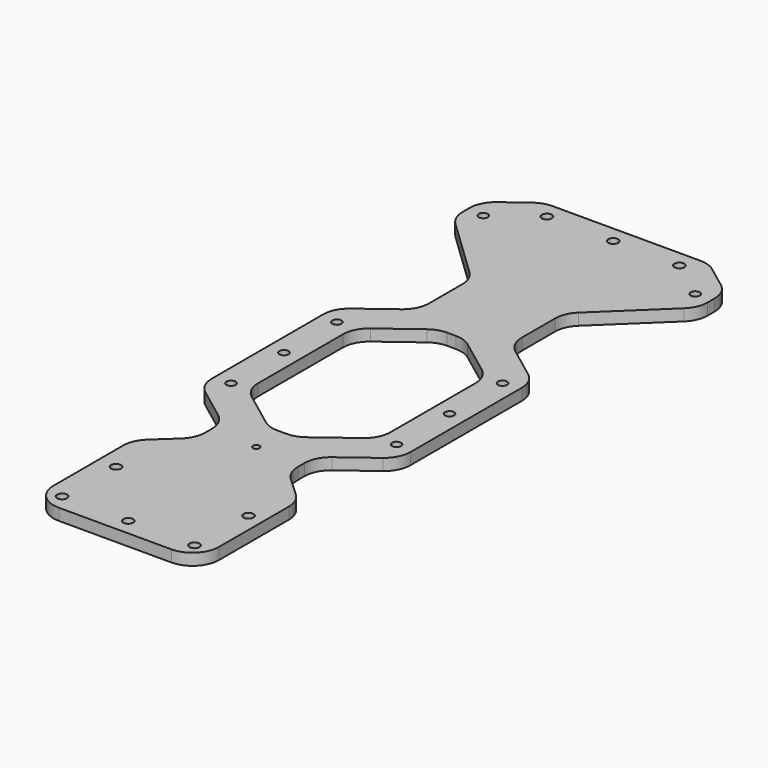
from build123d import *

# Parameters (mm, degrees)
F0_R     = 1.5
F0_R_2   = 1.375
F0_R_3   = 1
F1_DEPTH = 3.5
F2_R     = 8


# Not quite as in the source:
# - a feature names something its author has since deleted; it is built from what else it names


with BuildPart() as f1:
    # F0 (on Top) → F1 (new body)
    with BuildSketch(Plane.XY):
        Polygon((-37, 91), (-37, 81), (-14, 59), (-14, 39), (-30, 27), (-30, -23), (-14, -35), (-14, -45), (-25, -55.1980390272), (-25, -93), (25, -93), (25, -55.1980390272), (14, -45), (14, -35), (30, -23), (30, 27), (14, 39), (14, 59), (37, 81), (37, 91), (25, 100), (-25, 100), align=None)
        with Locations((-20, -88)):
            Circle(F0_R, mode=Mode.SUBTRACT)
        with Locations((-19.5, -68.25)):
            Circle(F0_R, mode=Mode.SUBTRACT)
        with Locations((-25, -18)):
            Circle(F0_R_2, mode=Mode.SUBTRACT)
        with Locations((-25, 2)):
            Circle(F0_R_2, mode=Mode.SUBTRACT)
        with Locations((0, -88)):
            Circle(F0_R, mode=Mode.SUBTRACT)
        with Locations((20, -88)):
            Circle(F0_R, mode=Mode.SUBTRACT)
        with Locations((20.5, -68.25)):
            Circle(F0_R, mode=Mode.SUBTRACT)
        with Locations((25, -18)):
            Circle(F0_R_2, mode=Mode.SUBTRACT)
        with Locations((25, 2)):
            Circle(F0_R_2, mode=Mode.SUBTRACT)
        with Locations((-25, 22)):
            Circle(F0_R_2, mode=Mode.SUBTRACT)
        with Locations((-32, 86)):
            Circle(F0_R_2, mode=Mode.SUBTRACT)
        with Locations((-20, 95)):
            Circle(F0_R, mode=Mode.SUBTRACT)
        Polygon((27, 86), (27, 85.2728960546), (4, 63.2728960546), (4, 34), (20, 22), (20, -18), (4, -30), (4, -49.3654190662), (15, -59.5634580934), (15, -83), (-15, -83), (-15, -59.5634580934), (-4, -49.3654190662), (-4, -30), (-20, -18), (-20, 22), (-4, 34), (-4, 63.2728960546), (-27, 85.2728960546), (-27, 86), (-21.6666666667, 90), (21.6666666667, 90), align=None, mode=Mode.SUBTRACT)
        with Locations((25, 22)):
            Circle(F0_R_2, mode=Mode.SUBTRACT)
        with Locations((0, 95)):
            Circle(F0_R, mode=Mode.SUBTRACT)
        with Locations((20, 95)):
            Circle(F0_R, mode=Mode.SUBTRACT)
        with Locations((32, 86)):
            Circle(F0_R_2, mode=Mode.SUBTRACT)
        Polygon((4, 63.2728960546), (27, 85.2728960546), (27, 86), (21.6666666667, 90), (-21.6666666667, 90), (-27, 86), (-27, 85.2728960546), (-4, 63.2728960546), (-4, 34), (4, 34), align=None)
        Polygon((4, -49.3654190662), (4, -30), (-4, -30), (-4, -49.3654190662), (-15, -59.5634580934), (-15, -83), (15, -83), (15, -59.5634580934), align=None)
        with Locations((0, -39.6827095331)):
            Circle(F0_R_3, mode=Mode.SUBTRACT)
    extrude(amount=F1_DEPTH)

    # F2
    f2_edges = [f1.edges().sort_by_distance(p)[0] for p in [
        (4, -30, 1.75),
        (-4, -30, 1.75),
        (20, -18, 1.75),
        (-25, -93, 1.75),
        (25, -93, 1.75),
        (25, -55.198039, 1.75),
        (14, -45, 1.75),
        (-25, -55.198039, 1.75),
        (-14, -45, 1.75),
        (-14, -35, 1.75),
        (14, -35, 1.75),
        (30, -23, 1.75),
        (-30, -23, 1.75),
        (-20, -18, 1.75),
        (-20, 22, 1.75),
        (20, 22, 1.75),
        (4, 34, 1.75),
        (-4, 34, 1.75),
        (-30, 27, 1.75),
        (-14, 39, 1.75),
        (30, 27, 1.75),
        (14, 39, 1.75),
        (-14, 59, 1.75),
        (14, 59, 1.75),
        (37, 81, 1.75),
        (37, 91, 1.75),
        (25, 100, 1.75),
        (-25, 100, 1.75),
        (-37, 81, 1.75),
        (-37, 91, 1.75),
    ]]
    fillet(f2_edges, radius=F2_R)


solid = f1.part
